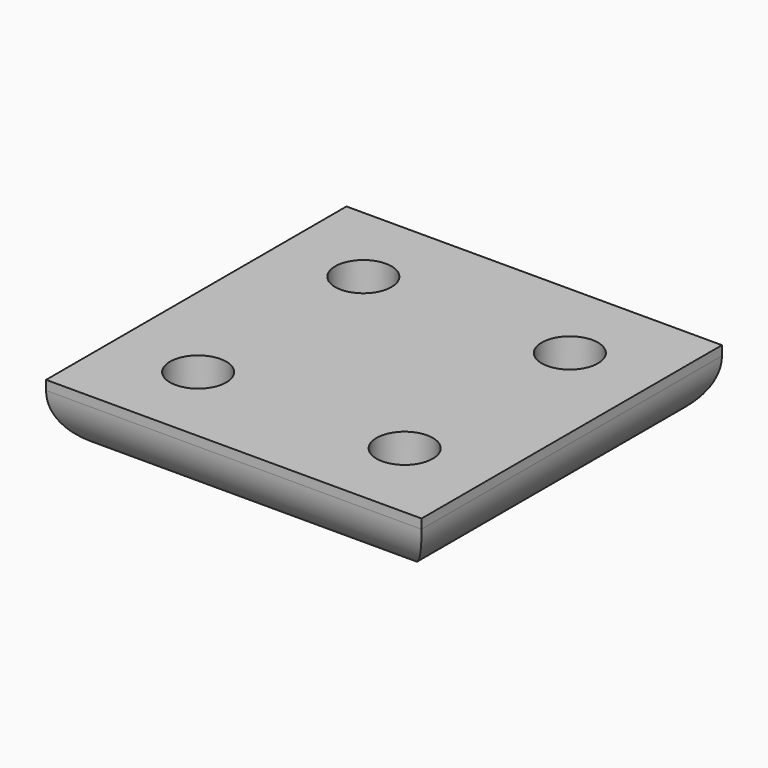
from build123d import *

# Parameters (mm, degrees)
F0_W     = 40
F0_H     = 40
F0_R     = 3
F1_DEPTH = 7
F2_R     = 5.99999


# Not quite as in the source:
# - a fillet or chamfer is up to 0.001 mm smaller than in the source, because OpenCascade refuses the exact size


with BuildPart() as f1:
    # F0 (on Top) → F1 (new body)
    with BuildSketch(Plane.XY):
        with Locations((20, 20)):
            Rectangle(F0_W, F0_H)
        with Locations((9, 9)):
            Circle(F0_R, mode=Mode.SUBTRACT)
        with Locations((31, 9)):
            Circle(F0_R, mode=Mode.SUBTRACT)
        with Locations((9, 31)):
            Circle(F0_R, mode=Mode.SUBTRACT)
        with Locations((31, 31)):
            Circle(F0_R, mode=Mode.SUBTRACT)
    extrude(amount=F1_DEPTH)

    # F2 (radius 6 in the source; OpenCascade refuses exactly that, so slightly less here)
    f2_edges = [f1.edges().sort_by_distance(p)[0] for p in [
        (40, 20, 0),
        (20, 0, 0),
        (0, 20, 0),
        (20, 40, 0),
    ]]
    fillet(f2_edges, radius=F2_R)


solid = f1.part
